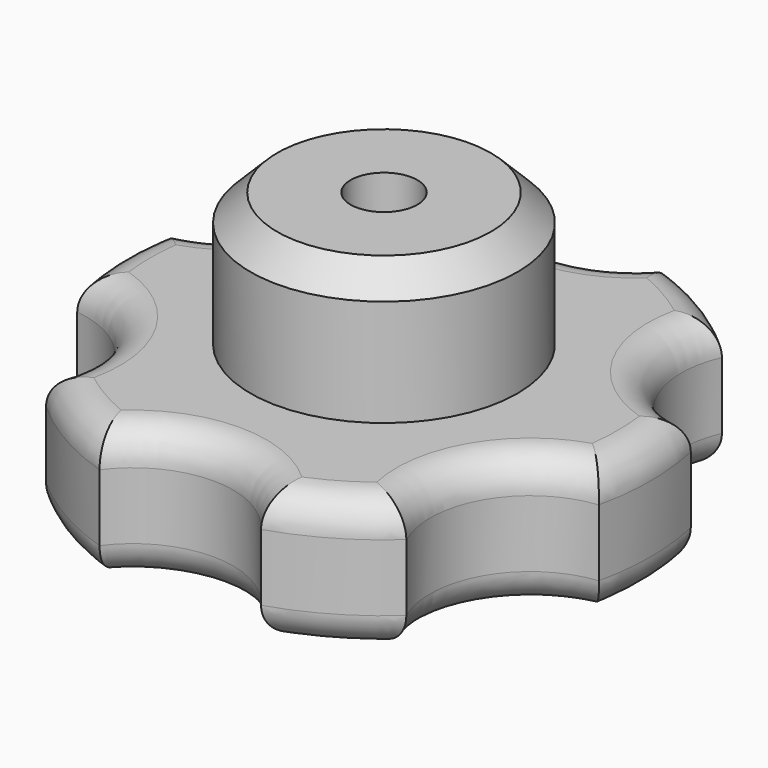
from build123d import *

# Parameters (mm, degrees)
F3_SIZE         = 4
F5_D            = 10
F5_DEPTH        = 25
F5_TIP          = 3.0043030951
F1_R            = 15
F6_DEPTH        = 40.001
F6_COPIES_COUNT = 6
F7_R            = 5
F8_R            = 4
F9_DEPTH        = 38.1286596745


# Not quite as in the source:
# - a pattern or mirror of a feature is missing from the dataset's text; its kind, count and spacing are read off the source's solid


with BuildPart() as f2:
    # F0 (on Front) → F2 (revolve)
    with BuildSketch(Plane.XZ):
        Polygon((0, 40), (0, 0), (40, 0), (40, 20), (20, 20), (20, 40), align=None)
    revolve(axis=Axis((0, 0, 20), (0, 0, -1)))

    # F3
    f3_edges = [f2.edges().sort_by_distance(p)[0] for p in [
        (-20, 0, 40),
    ]]
    chamfer(f3_edges, length=F3_SIZE)

    # F5
    with Locations(Plane.XY.offset(40)):
        with Locations((0, 0)):
            Hole(F5_D / 2, depth=F5_DEPTH)
            with Locations((0, 0, -(F5_DEPTH + F5_TIP / 2))):  # 118° drill point
                Cone(0, F5_D / 2, F5_TIP, mode=Mode.SUBTRACT)

    # F1 (on Top) → F6 (cut, through all)
    with BuildSketch(Plane.XY):
        with Locations((0, 47)):
            Circle(F1_R)
    f6 = extrude(amount=F6_DEPTH, mode=Mode.SUBTRACT)

    # F6_copies: F6 ×6 about axis
    f6_copies_axis = Axis((0, 0, 0), (0, 0, 1))
    for i in range(1, F6_COPIES_COUNT):
        add(f6.rotate(f6_copies_axis, i * 360 / F6_COPIES_COUNT), mode=Mode.SUBTRACT)

    # F7
    f7_edges = [f2.edges().sort_by_distance(p)[0] for p in [
        (-20, 34.641016, 20),
        (-40, 0, 20),
        (-20, -34.641016, 20),
        (20, -34.641016, 20),
        (40, 0, 20),
        (20, 34.641016, 20),
        (-20, 34.641016, 0),
        (-40, 0, 0),
        (-20, -34.641016, 0),
        (20, -34.641016, 0),
        (40, 0, 0),
        (20, 34.641016, 0),
        (0, 32, 0),
        (0, 32, 20),
        (-27.712813, 16, 20),
        (-27.712813, -16, 20),
        (0, -32, 20),
        (27.712813, -16, 20),
        (27.712813, 16, 20),
        (-27.712813, 16, 0),
        (-27.712813, -16, 0),
        (0, -32, 0),
        (27.712813, -16, 0),
        (27.712813, 16, 0),
    ]]
    fillet(f7_edges, radius=F7_R)

    # F8 (on Front) → F9 (cut, through all)
    with BuildSketch(Plane.XZ):
        with Locations((0, 30)):
            Circle(F8_R)
    extrude(amount=-F9_DEPTH, mode=Mode.SUBTRACT)


solid = f2.part
